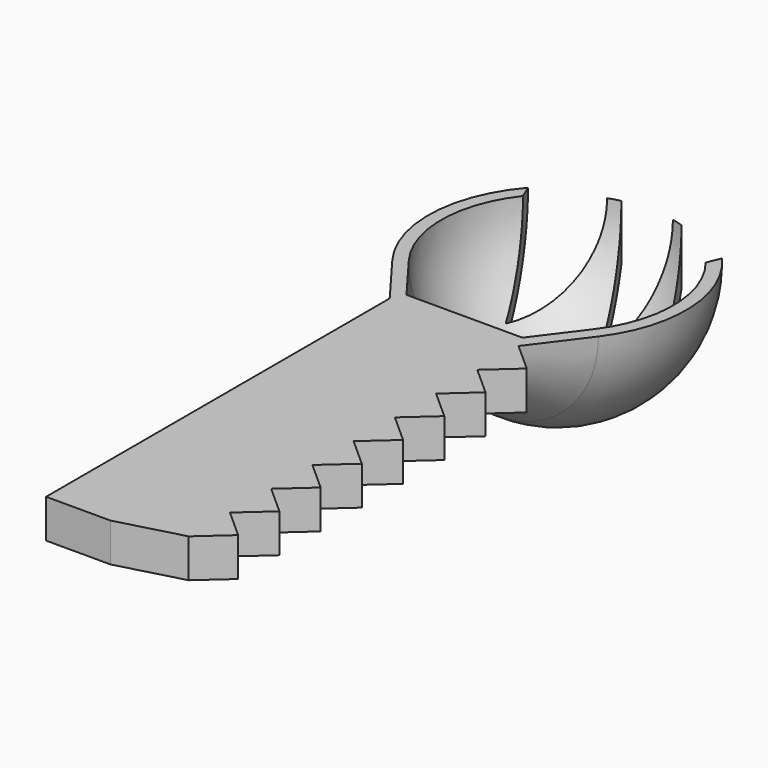
from build123d import *

# Parameters (mm, degrees)
F0_W     = 6.35
F0_H     = 42.3414773719
F1_DEPTH = 3.81
F3_ANGLE = 180
F4_T     = -1.27
F7_DEPTH = 25.4


# Not quite as in the source:
# - a feature names something its author has since deleted; it is built from what else it names


with BuildPart() as f1:
    # F0 (on Top) → F1 (new body)
    with BuildSketch(Plane.XY):
        Polygon((6.35, -30.48), (6.35, -35.56), (9.1898063314, -33.02), align=None)
        Polygon((6.35, -35.56), (6.35, -40.64), (9.1898063314, -38.1), align=None)
        Polygon((6.35, -25.4), (6.35, -30.48), (9.1898063314, -27.94), align=None)
        Polygon((6.35, -20.32), (6.35, -25.4), (9.1898063314, -22.86), align=None)
        Polygon((9.1898063314, -17.78), (6.35, -15.24), (6.35, -20.32), align=None)
        Polygon((9.1898063314, -12.7), (6.35, -10.16), (6.35, -15.24), align=None)
        Polygon((9.1898063314, -7.62), (6.35, -5.08), (6.35, -10.16), align=None)
        Polygon((9.1898063314, -2.54), (6.35, 0), (6.35, -5.08), align=None)
        Polygon((6.35, 0), (0, 0), (0, -42.3414773719), (6.35, -40.64), (6.35, -35.56), (6.35, -30.48), (6.35, -25.4), (6.35, -20.32), (6.35, -15.24), (6.35, -10.16), (6.35, -5.08), align=None)
        with Locations((-3.175, -21.170738686)):
            Rectangle(F0_W, F0_H)
    extrude(amount=F1_DEPTH)


with BuildPart() as f3:
    # F2 (on face) → F3 (revolve)
    with BuildSketch(Plane.XY.offset(3.81)):
        with BuildLine():
            ThreePointArc((10.16, 5.08), (5.6796126628, 1.3407746743), (0, 0))
            Line((0, 0), (6.35, 0))
            Line((6.35, 0), (10.16, 5.08))
        make_face()
        with BuildLine():
            Line((0, 25.4), (0, 0))
            ThreePointArc((0, 0), (5.6796126628, 1.3407746743), (10.16, 5.08))
            ThreePointArc((10.16, 5.08), (11.3592253257, 18.3796126628), (0, 25.4))
        make_face()
    revolve(axis=Axis((0, 12.7, 3.81), (0, 1, 0)), revolution_arc=F3_ANGLE)

    # F4
    f4_openings = [f3.faces().sort_by_distance(p)[0] for p in [
        (0, 12.436594, 3.81),
    ]]
    offset(amount=F4_T, openings=f4_openings)


with BuildPart() as f1_1:
    add(f1.part)

    # F5: union F3
    add(f3.part)

    # F6 (on face) → F7 (cut)
    with BuildSketch(Plane.XY.offset(3.81)):
        with BuildLine():
            Line((8.9097454996, 19.8597021678), (9.4470019608, 21.1878827721))
            ThreePointArc((9.4470019608, 21.1878827721), (5.1717448117, 24.299269615), (0, 25.4))
            ThreePointArc((0, 25.4), (-1.5546529222, 25.304485483), (-3.0859212896, 25.0193786286))
            Line((-3.0859212896, 25.0193786286), (-2.5834265714, 23.8342178508))
            ThreePointArc((-2.5834265714, 23.8342178508), (-1.3001519074, 24.0558137101), (0, 24.13))
            ThreePointArc((0, 24.13), (1.2447495309, 24.0620200055), (2.4746927509, 23.8588886449))
            Line((2.4746927509, 23.8588886449), (2.9447663441, 25.0209828664))
            Line((2.9447663441, 25.0209828664), (3.5641672216, 23.5600926339))
            ThreePointArc((3.5641672216, 23.5600926339), (6.5056012054, 22.0979813234), (8.9097454996, 19.8597021678))
        make_face()
        with BuildLine():
            Line((7.0658245088, 15.3012458764), (8.9097454996, 19.8597021678))
            ThreePointArc((8.9097454996, 19.8597021678), (6.5056012054, 22.0979813234), (3.5641672216, 23.5600926339))
            Line((3.5641672216, 23.5600926339), (7.0658245088, 15.3012458764))
        make_face()
        with BuildLine():
            ThreePointArc((2.4746927509, 23.8588886449), (3.0231237497, 23.7229588947), (3.5641672216, 23.5600926339))
            Line((3.5641672216, 23.5600926339), (2.9447663441, 25.0209828664))
            Line((2.9447663441, 25.0209828664), (2.4746927509, 23.8588886449))
        make_face()
        with BuildLine():
            Line((-2.5834265714, 23.8342178508), (-3.0859212896, 25.0193786286))
            ThreePointArc((-3.0859212896, 25.0193786286), (-3.1028243507, 25.0151321978), (-3.1197215685, 25.0108625748))
            Line((-3.1197215685, 25.0108625748), (-3.7290136249, 23.5045988998))
            ThreePointArc((-3.7290136249, 23.5045988998), (-3.1605201267, 23.6843530774), (-2.5834265714, 23.8342178508))
        make_face()
        with BuildLine():
            Line((0, 17.7410675473), (2.4746927509, 23.8588886449))
            ThreePointArc((2.4746927509, 23.8588886449), (1.2447495309, 24.0620200055), (0, 24.13))
            ThreePointArc((0, 24.13), (-1.3001519074, 24.0558137101), (-2.5834265714, 23.8342178508))
            Line((-2.5834265714, 23.8342178508), (0, 17.7410675473))
        make_face()
        with BuildLine():
            Line((-3.7290136249, 23.5045988998), (-3.1197215685, 25.0108625748))
            ThreePointArc((-3.1197215685, 25.0108625748), (-6.6419627447, 23.5247092754), (-9.562361361, 21.0577057379))
            Line((-9.562361361, 21.0577057379), (-9.0040057437, 19.7407940296))
            ThreePointArc((-9.0040057437, 19.7407940296), (-6.6388253732, 22.0043483202), (-3.7290136249, 23.5045988998))
        make_face()
        with BuildLine():
            Line((-7.0836272172, 15.211478147), (-3.7290136249, 23.5045988998))
            ThreePointArc((-3.7290136249, 23.5045988998), (-6.6388253732, 22.0043483202), (-9.0040057437, 19.7407940296))
            Line((-9.0040057437, 19.7407940296), (-7.0836272172, 15.211478147))
        make_face()
    extrude(amount=-F7_DEPTH, mode=Mode.SUBTRACT)


solid = f1_1.part
